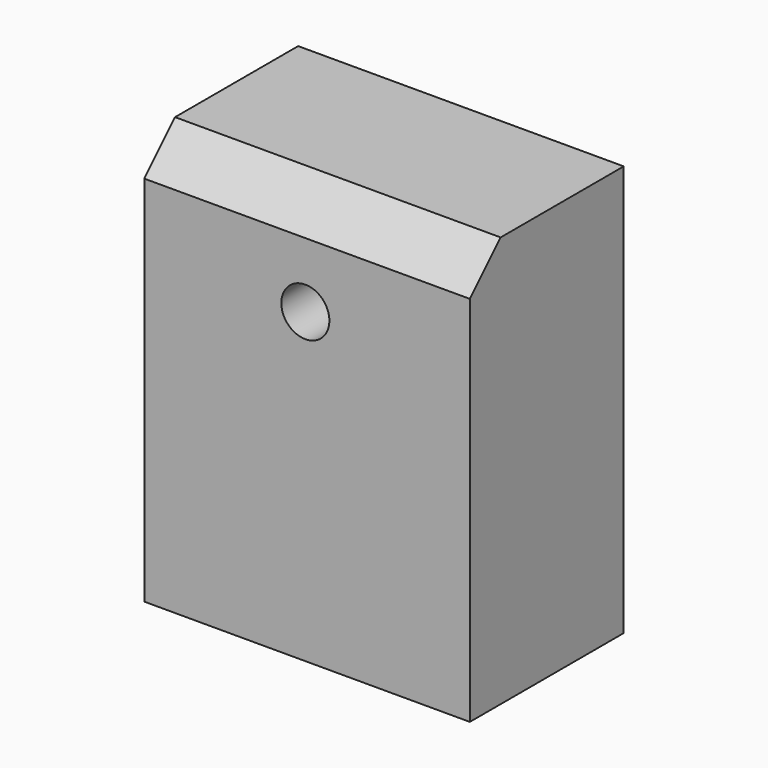
from build123d import *

# Parameters (mm, degrees)
F0_W     = 42.9938789457
F0_H     = 54.2596541345
F1_DEPTH = 25.4
F3_D     = 6.35
F6_SIZE  = 5.08


# Not quite as in the source:
# - the program builds the solid bodies; features that only make, move or delete a surface that nothing else refers to are left out


with BuildPart() as f1:
    # F0 (on Front) → F1 (new body)
    with BuildSketch(Plane.XZ):
        with Locations((8.1619387493, -0.9196549654)):
            Rectangle(F0_W, F0_H)
    extrude(amount=F1_DEPTH)

    # F3 (through all)
    with Locations(Plane.XZ.offset(25.4)):
        with Locations((7.9346429557, 12.5517835841)):
            Hole(F3_D / 2)

    # F6
    f6_edges = [f1.edges().sort_by_distance(p)[0] for p in [
        (8.161939, -25.4, 26.210172),
    ]]
    chamfer(f6_edges, length=F6_SIZE)


solid = f1.part
